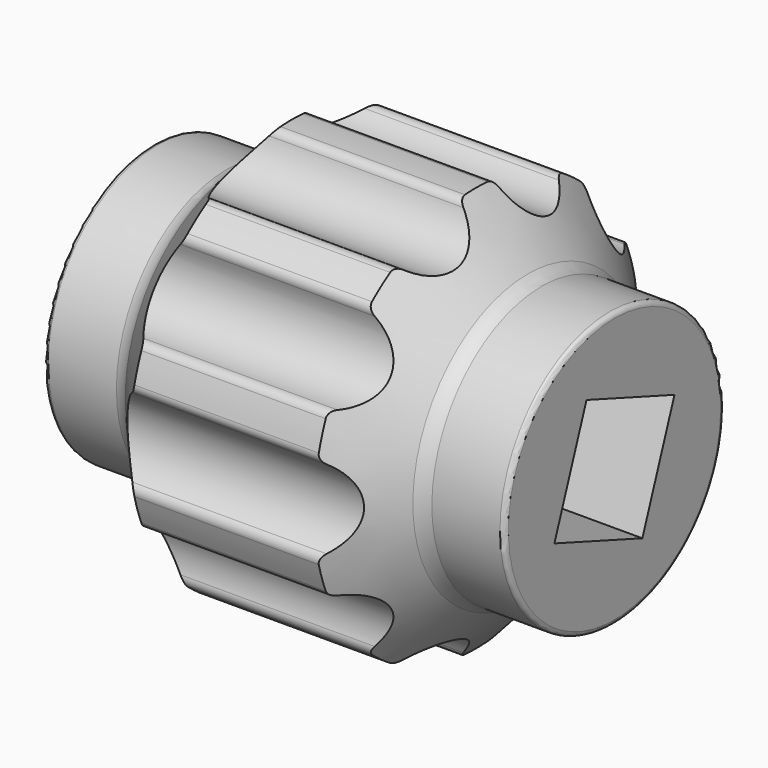
from build123d import *

# Parameters (mm, degrees)
F3_R        = 0.5
F2_R        = 5
F4_DEPTH    = 50
F2_R_2      = 5.25
F5_DEPTH    = 50
F6_R        = 2
F7_T1_DEPTH = 23.6514801136


# Not quite as in the source:
# - a fillet or chamfer that OpenCascade refuses, or shapes differently, is made with other operations: its cross-section is extruded or revolved along the edge and cut away or added
# - two fillets or chamfers of one size are made in one step


with BuildPart() as f1:
    # F0 (on Front) → F1 (revolve)
    with BuildSketch(Plane.XZ):
        Polygon((-27, 5), (23, 5), (23, 14.9), (14.2, 14.9), (8, 22), (-12, 22), (-18.2, 14.9), (-27, 14.9), align=None)
    revolve(axis=Axis((1.6108596474, 0, 0), (1, 0, 0)))

    # F3
    f3_edges = [f1.edges().sort_by_distance(p)[0] for p in [
        (-27, 0, -14.9),
        (23, 0, -14.9),
    ]]
    fillet(f3_edges, radius=F3_R)

    # F2 (on face) → F4 (cut)
    with BuildSketch(Plane.YZ.offset(23)):
        Polygon((3.7870547807, -8.1426786801), (8.1426786801, 3.7870547807), (-3.7870547807, 8.1426786801), (-8.1426786801, -3.7870547807), align=None)
        Circle(F2_R, mode=Mode.SUBTRACT)
    extrude(amount=-F4_DEPTH, mode=Mode.SUBTRACT)

    # F2 (on face) → F5 (cut)
    with BuildSketch(Plane.YZ.offset(23)):
        with Locations((19.416407865, 14.106846055)):
            Circle(F2_R_2)
        with Locations((24, 0)):
            Circle(F2_R_2)
        with Locations((19.416407865, -14.106846055)):
            Circle(F2_R_2)
        with Locations((7.416407865, -22.8253563911)):
            Circle(F2_R_2)
        with Locations((-7.416407865, -22.8253563911)):
            Circle(F2_R_2)
        with Locations((-19.416407865, -14.106846055)):
            Circle(F2_R_2)
        with Locations((-24, 0)):
            Circle(F2_R_2)
        with Locations((-7.416407865, 22.8253563911)):
            Circle(F2_R_2)
        with Locations((7.416407865, 22.8253563911)):
            Circle(F2_R_2)
        with Locations((-19.416407865, 14.106846055)):
            Circle(F2_R_2)
    extrude(amount=-F5_DEPTH, mode=Mode.SUBTRACT)

    # F6
    f6_edges = [f1.edges().sort_by_distance(p)[0] for p in [
        (-18.2, 0, -14.9),
        (14.2, 0, -14.9),
    ]]
    fillet(f6_edges, radius=F6_R)

    # F7: fillet of radius 1 on 20 edges, made by hand

    # F7_s2 → F7_t1 (cut)
    with BuildSketch(Plane.YZ.offset(-13.8257400568)):
        with BuildLine():
            ThreePointArc((10.5417904096, 18.6070055345), (11.0977849002, 18.8027369419), (11.667439531, 18.65129633))
            ThreePointArc((11.667439531, 18.65129633), (11.3562648943, 18.8423790337), (11.0419616007, 19.0282706521))
            ThreePointArc((11.0419616007, 19.0282706521), (10.7984414604, 18.8098428797), (10.5417904096, 18.6070055345))
        make_face()
        with BuildLine():
            ThreePointArc((1.5238000575, 21.9471645865), (2.073674893, 21.7348480242), (2.4084358499, 21.2496926273))
            ThreePointArc((2.4084358499, 21.2496926273), (2.3200255884, 21.5646471894), (2.2514022797, 21.8844965164))
            ThreePointArc((2.2514022797, 21.8844965164), (1.887861222, 21.9188498787), (1.5238000575, 21.9471645865))
        make_face()
        with BuildLine():
            ThreePointArc((-10.5417904096, 18.6070055345), (-11.0977849002, 18.8027369419), (-11.667439531, 18.65129633))
            ThreePointArc((-11.667439531, 18.65129633), (-11.3562648943, 18.8423790337), (-11.0419616007, 19.0282706521))
            ThreePointArc((-11.0419616007, 19.0282706521), (-10.7984414604, 18.8098428797), (-10.5417904096, 18.6070055345))
        make_face()
        with BuildLine():
            ThreePointArc((-1.5238000575, 21.9471645865), (-2.073674893, 21.7348480242), (-2.4084358499, 21.2496926273))
            ThreePointArc((-2.4084358499, 21.2496926273), (-2.3200255884, 21.5646471894), (-2.2514022797, 21.8844965164))
            ThreePointArc((-2.2514022797, 21.8844965164), (-1.887861222, 21.9188498787), (-1.5238000575, 21.9471645865))
        make_face()
        with BuildLine():
            ThreePointArc((14.1329998161, 16.8599619276), (14.4530613587, 16.3649859016), (14.4387214746, 15.7757193871))
            ThreePointArc((14.4387214746, 15.7757193871), (14.5523217172, 16.0824892281), (14.6848070116, 16.3815885381))
            ThreePointArc((14.6848070116, 16.3815885381), (14.4108885175, 16.6230650644), (14.1329998161, 16.8599619276))
        make_face()
        with BuildLine():
            ThreePointArc((19.465411035, 8.8570747563), (20.0302680613, 8.6886194293), (20.4021137804, 8.2312668097))
            ThreePointArc((20.4021137804, 8.2312668097), (20.2626838063, 8.5687598267), (20.1176714521, 8.9038921458))
            ThreePointArc((20.1176714521, 8.9038921458), (19.7922708968, 8.8703179131), (19.465411035, 8.8570747563))
        make_face()
        with BuildLine():
            ThreePointArc((21.3438740079, 5.3328268614), (21.3118696268, 4.74425539), (20.95390625, 4.2759575379))
            ThreePointArc((20.95390625, 4.2759575379), (21.2261255653, 4.4573670054), (21.5091145833, 4.621470528))
            ThreePointArc((21.5091145833, 4.621470528), (21.4294462075, 4.9778343927), (21.3438740079, 5.3328268614))
        make_face()
        with BuildLine():
            ThreePointArc((20.95390625, -4.2759575379), (21.3118696268, -4.74425539), (21.3438740079, -5.3328268614))
            ThreePointArc((21.3438740079, -5.3328268614), (21.4294462075, -4.9778343927), (21.5091145833, -4.621470528))
            ThreePointArc((21.5091145833, -4.621470528), (21.2261255653, -4.4573670054), (20.95390625, -4.2759575379))
        make_face()
        with BuildLine():
            ThreePointArc((20.4021137804, -8.2312668097), (20.0302680613, -8.6886194293), (19.465411035, -8.8570747563))
            ThreePointArc((19.465411035, -8.8570747563), (19.7922708968, -8.8703179131), (20.1176714521, -8.9038921458))
            ThreePointArc((20.1176714521, -8.9038921458), (20.2626838063, -8.5687598267), (20.4021137804, -8.2312668097))
        make_face()
        with BuildLine():
            ThreePointArc((14.4387214746, -15.7757193871), (14.4530613587, -16.3649859016), (14.1329998161, -16.8599619276))
            ThreePointArc((14.1329998161, -16.8599619276), (14.4108885175, -16.6230650644), (14.6848070116, -16.3815885381))
            ThreePointArc((14.6848070116, -16.3815885381), (14.5523217172, -16.0824892281), (14.4387214746, -15.7757193871))
        make_face()
        with BuildLine():
            ThreePointArc((11.667439531, -18.65129633), (11.0977849002, -18.8027369419), (10.5417904096, -18.6070055345))
            ThreePointArc((10.5417904096, -18.6070055345), (10.7984414604, -18.8098428797), (11.0419616007, -19.0282706521))
            ThreePointArc((11.0419616007, -19.0282706521), (11.3562648943, -18.8423790337), (11.667439531, -18.65129633))
        make_face()
        with BuildLine():
            ThreePointArc((1.5238000575, -21.9471645865), (2.073674893, -21.7348480242), (2.4084358499, -21.2496926273))
            ThreePointArc((2.4084358499, -21.2496926273), (2.3200255884, -21.5646471894), (2.2514022797, -21.8844965164))
            ThreePointArc((2.2514022797, -21.8844965164), (1.887861222, -21.9188498787), (1.5238000575, -21.9471645865))
        make_face()
        with BuildLine():
            ThreePointArc((-2.4084358499, -21.2496926273), (-2.073674893, -21.7348480242), (-1.5238000575, -21.9471645865))
            ThreePointArc((-1.5238000575, -21.9471645865), (-1.887861222, -21.9188498787), (-2.2514022797, -21.8844965164))
            ThreePointArc((-2.2514022797, -21.8844965164), (-2.3200255884, -21.5646471894), (-2.4084358499, -21.2496926273))
        make_face()
        with BuildLine():
            ThreePointArc((-11.667439531, -18.65129633), (-11.0977849002, -18.8027369419), (-10.5417904096, -18.6070055345))
            ThreePointArc((-10.5417904096, -18.6070055345), (-10.7984414604, -18.8098428797), (-11.0419616007, -19.0282706521))
            ThreePointArc((-11.0419616007, -19.0282706521), (-11.3562648943, -18.8423790337), (-11.667439531, -18.65129633))
        make_face()
        with BuildLine():
            ThreePointArc((-14.4387214746, -15.7757193871), (-14.4530613587, -16.3649859016), (-14.1329998161, -16.8599619276))
            ThreePointArc((-14.1329998161, -16.8599619276), (-14.4108885175, -16.6230650644), (-14.6848070116, -16.3815885381))
            ThreePointArc((-14.6848070116, -16.3815885381), (-14.5523217172, -16.0824892281), (-14.4387214746, -15.7757193871))
        make_face()
        with BuildLine():
            ThreePointArc((-20.4021137804, -8.2312668097), (-20.0302680613, -8.6886194293), (-19.465411035, -8.8570747563))
            ThreePointArc((-19.465411035, -8.8570747563), (-19.7922708968, -8.8703179131), (-20.1176714521, -8.9038921458))
            ThreePointArc((-20.1176714521, -8.9038921458), (-20.2626838063, -8.5687598267), (-20.4021137804, -8.2312668097))
        make_face()
        with BuildLine():
            ThreePointArc((-20.95390625, -4.2759575379), (-21.3118696268, -4.74425539), (-21.3438740079, -5.3328268614))
            ThreePointArc((-21.3438740079, -5.3328268614), (-21.4294462075, -4.9778343927), (-21.5091145833, -4.621470528))
            ThreePointArc((-21.5091145833, -4.621470528), (-21.2261255653, -4.4573670054), (-20.95390625, -4.2759575379))
        make_face()
        with BuildLine():
            ThreePointArc((-21.3438740079, 5.3328268614), (-21.3118696268, 4.74425539), (-20.95390625, 4.2759575379))
            ThreePointArc((-20.95390625, 4.2759575379), (-21.2261255653, 4.4573670054), (-21.5091145833, 4.621470528))
            ThreePointArc((-21.5091145833, 4.621470528), (-21.4294462075, 4.9778343927), (-21.3438740079, 5.3328268614))
        make_face()
        with BuildLine():
            ThreePointArc((-19.465411035, 8.8570747563), (-20.0302680613, 8.6886194293), (-20.4021137804, 8.2312668097))
            ThreePointArc((-20.4021137804, 8.2312668097), (-20.2626838063, 8.5687598267), (-20.1176714521, 8.9038921458))
            ThreePointArc((-20.1176714521, 8.9038921458), (-19.7922708968, 8.8703179131), (-19.465411035, 8.8570747563))
        make_face()
        with BuildLine():
            ThreePointArc((-14.1329998161, 16.8599619276), (-14.4530613587, 16.3649859016), (-14.4387214746, 15.7757193871))
            ThreePointArc((-14.4387214746, 15.7757193871), (-14.5523217172, 16.0824892281), (-14.6848070116, 16.3815885381))
            ThreePointArc((-14.6848070116, 16.3815885381), (-14.4108885175, 16.6230650644), (-14.1329998161, 16.8599619276))
        make_face()
    extrude(amount=F7_T1_DEPTH, mode=Mode.SUBTRACT)


with BuildPart() as f9_1:
    # F9: copy of F1
    add(f1.part.moved(Location((0, 71.6, 0))))


solid = f1.part
